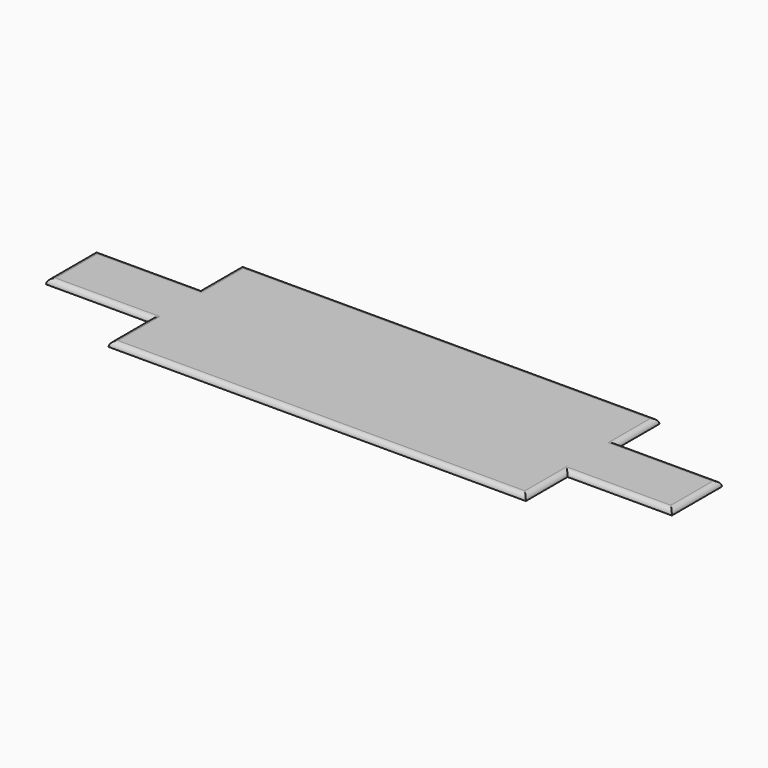
from build123d import *

# Parameters (mm, degrees)
F0_W     = 762
F0_H     = 203.2
F1_DEPTH = 6.35
F2_W     = 127
F2_H     = 63.5
F3_DEPTH = 25.4
F4_W     = 127
F4_H     = 63.5
F5_DEPTH = 25.4
F6_W     = 127
F6_H     = 63.5
F7_DEPTH = 25.4
F8_W     = 127
F8_H     = 63.5
F9_DEPTH = 25.4
F10_R    = 6.34999


# Not quite as in the source:
# - a fillet or chamfer is up to 0.001 mm smaller than in the source, because OpenCascade refuses the exact size


with BuildPart() as f1:
    # F0 (on Top) → F1 (new body)
    with BuildSketch(Plane.XY):
        Rectangle(F0_W, F0_H)
    extrude(amount=F1_DEPTH)

    # F2 (on face) → F3 (cut)
    with BuildSketch(Plane.XY.offset(6.35)):
        with Locations((317.5, 69.85)):
            Rectangle(F2_W, F2_H)
    extrude(amount=-F3_DEPTH, mode=Mode.SUBTRACT)

    # F4 (on face) → F5 (cut)
    with BuildSketch(Plane.XY.offset(6.35)):
        with Locations((317.5, -69.85)):
            Rectangle(F4_W, F4_H)
    extrude(amount=-F5_DEPTH, mode=Mode.SUBTRACT)

    # F6 (on face) → F7 (cut)
    with BuildSketch(Plane.XY.offset(6.35)):
        with Locations((-317.5, 69.85)):
            Rectangle(F6_W, F6_H)
    extrude(amount=-F7_DEPTH, mode=Mode.SUBTRACT)

    # F8 (on face) → F9 (cut)
    with BuildSketch(Plane.XY.offset(6.35)):
        with Locations((-317.5, -69.85)):
            Rectangle(F8_W, F8_H)
    extrude(amount=-F9_DEPTH, mode=Mode.SUBTRACT)

    # F10 (radius 6.35 in the source; OpenCascade refuses exactly that, so slightly less here)
    f10_edges = [f1.edges().sort_by_distance(p)[0] for p in [
        (-317.5, 38.1, 6.35),
        (-254, 69.85, 6.35),
        (0, 101.6, 6.35),
        (254, 69.85, 6.35),
        (317.5, 38.1, 6.35),
        (381, 0, 6.35),
        (317.5, -38.1, 6.35),
        (254, -69.85, 6.35),
        (0, -101.6, 6.35),
        (-254, -69.85, 6.35),
        (-317.5, -38.1, 6.35),
        (-381, 0, 6.35),
    ]]
    fillet(f10_edges, radius=F10_R)


solid = f1.part
